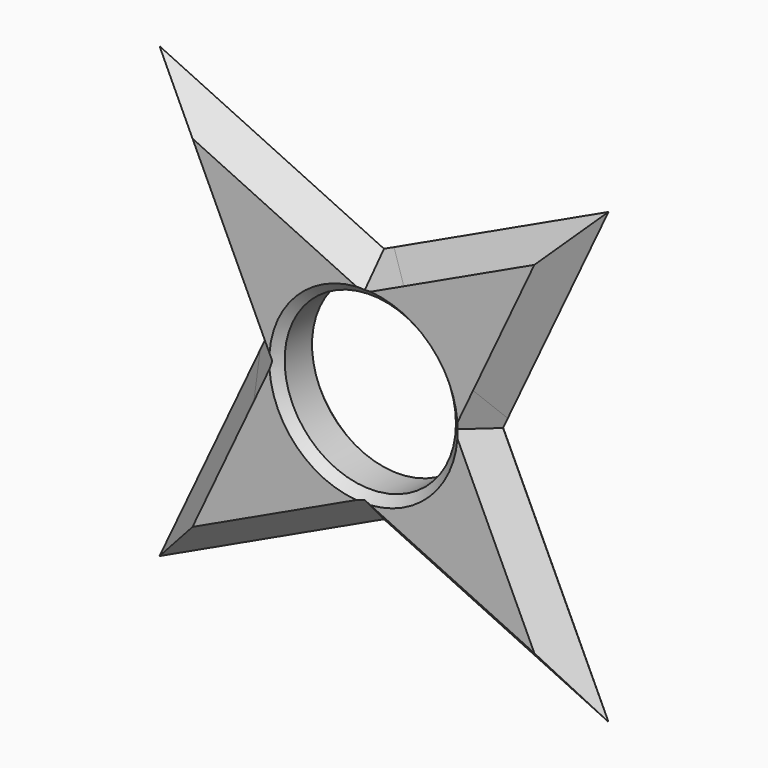
from build123d import *

# Parameters (mm, degrees)
F0_R          = 12.7
F1_DEPTH      = 7.62
F2_SIZE       = 1.27
F3_SIZE       = 1.27
F4_SIZE       = 5.08
F5_T4_DEPTH   = 65.8139573625
F6_SIZE       = 5.08
F7_T4_DEPTH   = 57.8584590231
F8_T4_DEPTH   = 72.4149723957
F8_T10_DEPTH  = 72.4149723957
F8_T16_DEPTH  = 72.4149723957
F9_T4_DEPTH   = 72.4149723957
F10_SIZE      = 5.08
F11_T4_DEPTH  = 57.8584590231
F12_T4_DEPTH  = 72.4149723957
F12_T10_DEPTH = 72.4149723957
F12_T16_DEPTH = 72.4149723957
F13_T4_DEPTH  = 72.4149723957
F14_SIZE      = 5.08
F15_T4_DEPTH  = 57.8584590231
F16_T4_DEPTH  = 72.4149723957
F16_T10_DEPTH = 72.4149723957
F16_T16_DEPTH = 72.4149723957
F17_T4_DEPTH  = 72.4149723957
F18_T4_DEPTH  = 64.4594740563
F18_T10_DEPTH = 64.4594740563
F18_T16_DEPTH = 64.4594740563
F19_T4_DEPTH  = 64.4594740563


# Not quite as in the source:
# - a fillet or chamfer that OpenCascade refuses, or shapes differently, is made with other operations: its cross-section is extruded or revolved along the edge and cut away or added


with BuildPart() as f1:
    # F0 (on Front) → F1 (new body)
    with BuildSketch(Plane.XZ):
        Polygon((-19.05, 0), (-35.9210244843, -35.9210244843), (0, -19.05), (35.9210244843, -35.9210244843), (19.05, 0), (35.9210244843, 35.9210244843), (0, 19.05), (-35.9210244843, 35.9210244843), align=None)
        Circle(F0_R, mode=Mode.SUBTRACT)
    extrude(amount=F1_DEPTH)

    # F2
    f2_edges = [f1.edges().sort_by_distance(p)[0] for p in [
        (-12.7, -7.62, 0),
    ]]
    chamfer(f2_edges, length=F2_SIZE)

    # F3
    f3_edges = [f1.edges().sort_by_distance(p)[0] for p in [
        (-12.7, 0, 0),
    ]]
    chamfer(f3_edges, length=F3_SIZE)

    # F4
    f4_edges = [f1.edges().sort_by_distance(p)[0] for p in [
        (17.960512, -7.62, 27.485512),
    ]]
    chamfer(f4_edges, length=F4_SIZE)

    # F5: chamfer of 5.08 on 1 edges, made by hand


with BuildPart() as f5_tool2:
    # F5_s3 → F5_t4 (new body)
    with BuildSketch(Plane(origin=(55.0761279539, 0, 25.8676002856), x_dir=(0, 1, 0), z_dir=(-0.9051386851, 0, -0.4251164085))):
        Polygon((-5.08, -17.2428919509), (0, -12.1628919509), (0, -17.2428919509), align=None)
    extrude(amount=F5_T4_DEPTH)

    split(bisect_by=Plane(origin=(7.330236298, 0, 15.6072085475), x_dir=(0, 1, 0), z_dir=(0.4251164085, 0, 0.9051386851)), keep=Keep.TOP)


with BuildPart() as f1_1:
    add(f1.part)

    # F5_t1: cut F5_tool2
    add(f5_tool2.part, mode=Mode.SUBTRACT)

    # F6
    f6_edges = [f1_1.edges().sort_by_distance(p)[0] for p in [
        (25.794506, -7.62, 14.360098),
    ]]
    chamfer(f6_edges, length=F6_SIZE)

    # F7: chamfer of 5.08 on 1 edges, made by hand


with BuildPart() as f7_tool2:
    # F7_s3 → F7_t4 (new body)
    with BuildSketch(Plane(origin=(-2.1109928963, 0, -4.4946308736), x_dir=(0, 1, 0), z_dir=(0.4251164085, 0, 0.9051386851))):
        Polygon((-5.08, -17.2428919509), (0, -12.1628919509), (0, -17.2428919509), align=None)
    extrude(amount=F7_T4_DEPTH)

    split(bisect_by=Plane(origin=(15.6072085475, 0, 7.330236298), x_dir=(0, 1, 0), z_dir=(0.9051386851, 0, 0.4251164085)), keep=Keep.TOP)


with BuildPart() as f1_2:
    add(f1_1.part)

    # F7_t1: cut F7_tool2
    add(f7_tool2.part, mode=Mode.SUBTRACT)

    # F8: chamfer of 5.08 on 1 edges, made by hand


with BuildPart() as f8_tool2:
    # F8_s3 → F8_t4 (new body)
    with BuildSketch(Plane(origin=(25.8676002856, 0, -55.0761279539), x_dir=(0, 1, 0), z_dir=(-0.4251164085, 0, 0.9051386851))):
        Polygon((-7.62, -12.1628919509), (-2.54, -17.2428919509), (-7.62, -17.2428919509), align=None)
    extrude(amount=F8_T4_DEPTH)

    split(bisect_by=Plane(origin=(5.5045520136, 6.0814459754, -2.5853224715), x_dir=(-0.741396788, 0.6710669138, 0), z_dir=(0.6400297021, 0.7071067812, -0.3006026952)), keep=Keep.TOP)

    split(bisect_by=Plane(origin=(8.9531304038, -9.8914459754, -4.2050159878), x_dir=(0.741396788, 0.6710669138, 0), z_dir=(0.6400297021, -0.7071067812, -0.3006026952)), keep=Keep.TOP)


with BuildPart() as f1_3:
    add(f1_2.part)

    # F8_t1: cut F8_tool2
    add(f8_tool2.part, mode=Mode.SUBTRACT)


with BuildPart() as f8_tool8:
    # F8_s9 → F8_t10 (new body)
    with BuildSketch(Plane(origin=(25.8676002856, 0, -55.0761279539), x_dir=(0, 1, 0), z_dir=(-0.4251164085, 0, 0.9051386851))):
        Polygon((-7.62, -12.1628919509), (-2.54, -17.2428919509), (-7.62, -17.2428919509), align=None)
    extrude(amount=F8_T10_DEPTH)

    split(bisect_by=Plane(origin=(5.5045520136, 6.0814459754, -2.5853224715), x_dir=(-0.741396788, 0.6710669138, 0), z_dir=(0.6400297021, 0.7071067812, -0.3006026952)), keep=Keep.TOP)

    split(bisect_by=Plane(origin=(8.9531304038, -9.8914459754, -4.2050159878), x_dir=(-0.741396788, -0.6710669138, 0), z_dir=(-0.6400297021, 0.7071067812, 0.3006026952)), keep=Keep.TOP)


with BuildPart() as f1_4:
    add(f1_3.part)

    # F8_t7: cut F8_tool8
    add(f8_tool8.part, mode=Mode.SUBTRACT)


with BuildPart() as f8_tool14:
    # F8_s15 → F8_t16 (new body)
    with BuildSketch(Plane(origin=(25.8676002856, 0, -55.0761279539), x_dir=(0, 1, 0), z_dir=(-0.4251164085, 0, 0.9051386851))):
        Polygon((-7.62, -12.1628919509), (-2.54, -17.2428919509), (-7.62, -17.2428919509), align=None)
    extrude(amount=F8_T16_DEPTH)

    split(bisect_by=Plane(origin=(5.5045520136, 6.0814459754, -2.5853224715), x_dir=(0.741396788, -0.6710669138, 0), z_dir=(-0.6400297021, -0.7071067812, 0.3006026952)), keep=Keep.TOP)

    split(bisect_by=Plane(origin=(8.9531304038, -9.8914459754, -4.2050159878), x_dir=(0.741396788, 0.6710669138, 0), z_dir=(0.6400297021, -0.7071067812, -0.3006026952)), keep=Keep.TOP)


with BuildPart() as f1_5:
    add(f1_4.part)

    # F8_t13: cut F8_tool14
    add(f8_tool14.part, mode=Mode.SUBTRACT)

    # F9: chamfer of 5.08 on 1 edges, made by hand


with BuildPart() as f9_tool2:
    # F9_s3 → F9_t4 (new body)
    with BuildSketch(Plane(origin=(25.8676002856, 0, -55.0761279539), x_dir=(0, 1, 0), z_dir=(-0.4251164085, 0, 0.9051386851))):
        Polygon((0, -12.1628919509), (-5.08, -17.2428919509), (0, -17.2428919509), align=None)
    extrude(amount=F9_T4_DEPTH)

    split(bisect_by=Plane(origin=(5.5045520136, 6.0814459754, -2.5853224715), x_dir=(-0.741396788, 0.6710669138, 0), z_dir=(0.6400297021, 0.7071067812, -0.3006026952)), keep=Keep.TOP)


with BuildPart() as f1_6:
    add(f1_5.part)

    # F9_t1: cut F9_tool2
    add(f9_tool2.part, mode=Mode.SUBTRACT)

    # F10
    f10_edges = [f1_6.edges().sort_by_distance(p)[0] for p in [
        (14.360098, -7.62, -25.794506),
    ]]
    chamfer(f10_edges, length=F10_SIZE)

    # F11: chamfer of 5.08 on 1 edges, made by hand


with BuildPart() as f11_tool2:
    # F11_s3 → F11_t4 (new body)
    with BuildSketch(Plane(origin=(-4.4946308736, 0, 2.1109928963), x_dir=(0, 1, 0), z_dir=(0.9051386851, 0, -0.4251164085))):
        Polygon((-5.08, -17.2428919509), (0, -12.1628919509), (0, -17.2428919509), align=None)
    extrude(amount=F11_T4_DEPTH)

    split(bisect_by=Plane(origin=(7.330236298, 0, -15.6072085475), x_dir=(0, 1, 0), z_dir=(0.4251164085, 0, -0.9051386851)), keep=Keep.TOP)


with BuildPart() as f1_7:
    add(f1_6.part)

    # F11_t1: cut F11_tool2
    add(f11_tool2.part, mode=Mode.SUBTRACT)

    # F12: chamfer of 5.08 on 1 edges, made by hand


with BuildPart() as f12_tool2:
    # F12_s3 → F12_t4 (new body)
    with BuildSketch(Plane(origin=(-55.0761279539, 0, -25.8676002856), x_dir=(0, 1, 0), z_dir=(0.9051386851, 0, 0.4251164085))):
        Polygon((0, -12.1628919509), (-5.08, -17.2428919509), (0, -17.2428919509), align=None)
    extrude(amount=F12_T4_DEPTH)

    split(bisect_by=Plane(origin=(-4.2050159878, -9.8914459754, -8.9531304038), x_dir=(0.9202923495, -0.3912313784, 0), z_dir=(-0.3006026952, -0.7071067812, -0.6400297021)), keep=Keep.TOP)

    split(bisect_by=Plane(origin=(-2.5853224715, 6.0814459755, -5.5045520136), x_dir=(-0.9202923495, -0.3912313784, 0), z_dir=(-0.3006026952, 0.7071067812, -0.6400297021)), keep=Keep.TOP)


with BuildPart() as f1_8:
    add(f1_7.part)

    # F12_t1: cut F12_tool2
    add(f12_tool2.part, mode=Mode.SUBTRACT)


with BuildPart() as f12_tool8:
    # F12_s9 → F12_t10 (new body)
    with BuildSketch(Plane(origin=(-55.0761279539, 0, -25.8676002856), x_dir=(0, 1, 0), z_dir=(0.9051386851, 0, 0.4251164085))):
        Polygon((0, -12.1628919509), (-5.08, -17.2428919509), (0, -17.2428919509), align=None)
    extrude(amount=F12_T10_DEPTH)

    split(bisect_by=Plane(origin=(-4.2050159878, -9.8914459754, -8.9531304038), x_dir=(0.9202923495, -0.3912313784, 0), z_dir=(-0.3006026952, -0.7071067812, -0.6400297021)), keep=Keep.TOP)

    split(bisect_by=Plane(origin=(-2.5853224715, 6.0814459755, -5.5045520136), x_dir=(0.9202923495, 0.3912313784, 0), z_dir=(0.3006026952, -0.7071067812, 0.6400297021)), keep=Keep.TOP)


with BuildPart() as f1_9:
    add(f1_8.part)

    # F12_t7: cut F12_tool8
    add(f12_tool8.part, mode=Mode.SUBTRACT)


with BuildPart() as f12_tool14:
    # F12_s15 → F12_t16 (new body)
    with BuildSketch(Plane(origin=(-55.0761279539, 0, -25.8676002856), x_dir=(0, 1, 0), z_dir=(0.9051386851, 0, 0.4251164085))):
        Polygon((0, -12.1628919509), (-5.08, -17.2428919509), (0, -17.2428919509), align=None)
    extrude(amount=F12_T16_DEPTH)

    split(bisect_by=Plane(origin=(-4.2050159878, -9.8914459754, -8.9531304038), x_dir=(-0.9202923495, 0.3912313784, 0), z_dir=(0.3006026952, 0.7071067812, 0.6400297021)), keep=Keep.TOP)

    split(bisect_by=Plane(origin=(-2.5853224715, 6.0814459755, -5.5045520136), x_dir=(-0.9202923495, -0.3912313784, 0), z_dir=(-0.3006026952, 0.7071067812, -0.6400297021)), keep=Keep.TOP)


with BuildPart() as f1_10:
    add(f1_9.part)

    # F12_t13: cut F12_tool14
    add(f12_tool14.part, mode=Mode.SUBTRACT)

    # F13: chamfer of 5.08 on 1 edges, made by hand


with BuildPart() as f13_tool2:
    # F13_s3 → F13_t4 (new body)
    with BuildSketch(Plane(origin=(-55.0761279539, 0, -25.8676002856), x_dir=(0, 1, 0), z_dir=(0.9051386851, 0, 0.4251164085))):
        Polygon((-7.62, -12.1628919509), (-2.54, -17.2428919509), (-7.62, -17.2428919509), align=None)
    extrude(amount=F13_T4_DEPTH)

    split(bisect_by=Plane(origin=(-4.2050159878, -9.8914459754, -8.9531304038), x_dir=(0.9202923495, -0.3912313784, 0), z_dir=(-0.3006026952, -0.7071067812, -0.6400297021)), keep=Keep.TOP)


with BuildPart() as f1_11:
    add(f1_10.part)

    # F13_t1: cut F13_tool2
    add(f13_tool2.part, mode=Mode.SUBTRACT)

    # F14
    f14_edges = [f1_11.edges().sort_by_distance(p)[0] for p in [
        (-25.794506, -7.62, -14.360098),
    ]]
    chamfer(f14_edges, length=F14_SIZE)

    # F15: chamfer of 5.08 on 1 edges, made by hand


with BuildPart() as f15_tool2:
    # F15_s3 → F15_t4 (new body)
    with BuildSketch(Plane(origin=(2.1109928963, 0, 4.4946308736), x_dir=(0, 1, 0), z_dir=(-0.4251164085, 0, -0.9051386851))):
        Polygon((-5.08, -17.2428919509), (0, -12.1628919509), (0, -17.2428919509), align=None)
    extrude(amount=F15_T4_DEPTH)

    split(bisect_by=Plane(origin=(-15.6072085475, 0, -7.330236298), x_dir=(0, 1, 0), z_dir=(-0.9051386851, 0, -0.4251164085)), keep=Keep.TOP)


with BuildPart() as f1_12:
    add(f1_11.part)

    # F15_t1: cut F15_tool2
    add(f15_tool2.part, mode=Mode.SUBTRACT)

    # F16: chamfer of 5.08 on 1 edges, made by hand


with BuildPart() as f16_tool2:
    # F16_s3 → F16_t4 (new body)
    with BuildSketch(Plane(origin=(-25.8676002856, 0, 55.0761279539), x_dir=(0, 1, 0), z_dir=(0.4251164085, 0, -0.9051386851))):
        Polygon((-7.62, -12.1628919509), (-2.54, -17.2428919509), (-7.62, -17.2428919509), align=None)
    extrude(amount=F16_T4_DEPTH)

    split(bisect_by=Plane(origin=(-5.5045520136, 6.0814459754, 2.5853224715), x_dir=(-0.741396788, -0.6710669138, 0), z_dir=(-0.6400297021, 0.7071067812, 0.3006026952)), keep=Keep.TOP)

    split(bisect_by=Plane(origin=(-8.9531304038, -9.8914459754, 4.2050159878), x_dir=(0.741396788, -0.6710669138, 0), z_dir=(-0.6400297021, -0.7071067812, 0.3006026952)), keep=Keep.TOP)


with BuildPart() as f1_13:
    add(f1_12.part)

    # F16_t1: cut F16_tool2
    add(f16_tool2.part, mode=Mode.SUBTRACT)


with BuildPart() as f16_tool8:
    # F16_s9 → F16_t10 (new body)
    with BuildSketch(Plane(origin=(-25.8676002856, 0, 55.0761279539), x_dir=(0, 1, 0), z_dir=(0.4251164085, 0, -0.9051386851))):
        Polygon((-7.62, -12.1628919509), (-2.54, -17.2428919509), (-7.62, -17.2428919509), align=None)
    extrude(amount=F16_T10_DEPTH)

    split(bisect_by=Plane(origin=(-5.5045520136, 6.0814459754, 2.5853224715), x_dir=(-0.741396788, -0.6710669138, 0), z_dir=(-0.6400297021, 0.7071067812, 0.3006026952)), keep=Keep.TOP)

    split(bisect_by=Plane(origin=(-8.9531304038, -9.8914459754, 4.2050159878), x_dir=(-0.741396788, 0.6710669138, 0), z_dir=(0.6400297021, 0.7071067812, -0.3006026952)), keep=Keep.TOP)


with BuildPart() as f1_14:
    add(f1_13.part)

    # F16_t7: cut F16_tool8
    add(f16_tool8.part, mode=Mode.SUBTRACT)


with BuildPart() as f16_tool14:
    # F16_s15 → F16_t16 (new body)
    with BuildSketch(Plane(origin=(-25.8676002856, 0, 55.0761279539), x_dir=(0, 1, 0), z_dir=(0.4251164085, 0, -0.9051386851))):
        Polygon((-7.62, -12.1628919509), (-2.54, -17.2428919509), (-7.62, -17.2428919509), align=None)
    extrude(amount=F16_T16_DEPTH)

    split(bisect_by=Plane(origin=(-5.5045520136, 6.0814459754, 2.5853224715), x_dir=(0.741396788, 0.6710669138, 0), z_dir=(0.6400297021, -0.7071067812, -0.3006026952)), keep=Keep.TOP)

    split(bisect_by=Plane(origin=(-8.9531304038, -9.8914459754, 4.2050159878), x_dir=(0.741396788, -0.6710669138, 0), z_dir=(-0.6400297021, -0.7071067812, 0.3006026952)), keep=Keep.TOP)


with BuildPart() as f1_15:
    add(f1_14.part)

    # F16_t13: cut F16_tool14
    add(f16_tool14.part, mode=Mode.SUBTRACT)

    # F17: chamfer of 5.08 on 1 edges, made by hand


with BuildPart() as f17_tool2:
    # F17_s3 → F17_t4 (new body)
    with BuildSketch(Plane(origin=(4.9171926996, 0, -10.4694649409), x_dir=(0, 1, 0), z_dir=(-0.4251164085, 0, 0.9051386851))):
        Polygon((-5.08, 17.2428919509), (0, 12.1628919509), (0, 17.2428919509), align=None)
    extrude(amount=F17_T4_DEPTH)

    split(bisect_by=Plane(origin=(-5.5045520136, 6.0814459754, 2.5853224715), x_dir=(-0.741396788, -0.6710669138, 0), z_dir=(-0.6400297021, 0.7071067812, 0.3006026952)), keep=Keep.TOP)


with BuildPart() as f1_16:
    add(f1_15.part)

    # F17_t1: cut F17_tool2
    add(f17_tool2.part, mode=Mode.SUBTRACT)

    # F18: chamfer of 5.08 on 1 edges, made by hand


with BuildPart() as f18_tool2:
    # F18_s3 → F18_t4 (new body)
    with BuildSketch(Plane(origin=(10.469464941, 0, -4.9171926996), x_dir=(0, 1, 0), z_dir=(-0.9051386851, 0, 0.4251164085))):
        Polygon((-2.54, -17.2428919509), (-7.62, -12.1628919509), (-7.62, -17.2428919509), align=None)
    extrude(amount=F18_T4_DEPTH)

    split(bisect_by=Plane(origin=(-4.2050159878, -9.8914459754, 8.9531304038), x_dir=(0.9202923495, -0.3912313784, 0), z_dir=(-0.3006026952, -0.7071067812, 0.6400297021)), keep=Keep.TOP)

    split(bisect_by=Plane(origin=(-2.5853224715, 6.0814459755, 5.5045520136), x_dir=(0.9202923495, 0.3912313784, 0), z_dir=(0.3006026952, -0.7071067812, -0.6400297021)), keep=Keep.TOP)


with BuildPart() as f1_17:
    add(f1_16.part)

    # F18_t1: cut F18_tool2
    add(f18_tool2.part, mode=Mode.SUBTRACT)


with BuildPart() as f18_tool8:
    # F18_s9 → F18_t10 (new body)
    with BuildSketch(Plane(origin=(10.469464941, 0, -4.9171926996), x_dir=(0, 1, 0), z_dir=(-0.9051386851, 0, 0.4251164085))):
        Polygon((-2.54, -17.2428919509), (-7.62, -12.1628919509), (-7.62, -17.2428919509), align=None)
    extrude(amount=F18_T10_DEPTH)

    split(bisect_by=Plane(origin=(-4.2050159878, -9.8914459754, 8.9531304038), x_dir=(-0.9202923495, 0.3912313784, 0), z_dir=(0.3006026952, 0.7071067812, -0.6400297021)), keep=Keep.TOP)

    split(bisect_by=Plane(origin=(-2.5853224715, 6.0814459755, 5.5045520136), x_dir=(-0.9202923495, -0.3912313784, 0), z_dir=(-0.3006026952, 0.7071067812, 0.6400297021)), keep=Keep.TOP)


with BuildPart() as f1_18:
    add(f1_17.part)

    # F18_t7: cut F18_tool8
    add(f18_tool8.part, mode=Mode.SUBTRACT)


with BuildPart() as f18_tool14:
    # F18_s15 → F18_t16 (new body)
    with BuildSketch(Plane(origin=(10.469464941, 0, -4.9171926996), x_dir=(0, 1, 0), z_dir=(-0.9051386851, 0, 0.4251164085))):
        Polygon((-2.54, -17.2428919509), (-7.62, -12.1628919509), (-7.62, -17.2428919509), align=None)
    extrude(amount=F18_T16_DEPTH)

    split(bisect_by=Plane(origin=(-4.2050159878, -9.8914459754, 8.9531304038), x_dir=(0.9202923495, -0.3912313784, 0), z_dir=(-0.3006026952, -0.7071067812, 0.6400297021)), keep=Keep.TOP)

    split(bisect_by=Plane(origin=(-2.5853224715, 6.0814459755, 5.5045520136), x_dir=(-0.9202923495, -0.3912313784, 0), z_dir=(-0.3006026952, 0.7071067812, 0.6400297021)), keep=Keep.TOP)


with BuildPart() as f1_19:
    add(f1_18.part)

    # F18_t13: cut F18_tool14
    add(f18_tool14.part, mode=Mode.SUBTRACT)

    # F19: chamfer of 5.08 on 1 edges, made by hand


with BuildPart() as f19_tool2:
    # F19_s3 → F19_t4 (new body)
    with BuildSketch(Plane(origin=(10.4694649409, 0, -4.9171926996), x_dir=(0, 1, 0), z_dir=(-0.9051386851, 0, 0.4251164085))):
        Polygon((-5.08, -17.2428919509), (0, -12.1628919509), (0, -17.2428919509), align=None)
    extrude(amount=F19_T4_DEPTH)

    split(bisect_by=Plane(origin=(-2.5853224715, 6.0814459755, 5.5045520136), x_dir=(-0.9202923495, -0.3912313784, 0), z_dir=(-0.3006026952, 0.7071067812, 0.6400297021)), keep=Keep.TOP)


with BuildPart() as f1_20:
    add(f1_19.part)

    # F19_t1: cut F19_tool2
    add(f19_tool2.part, mode=Mode.SUBTRACT)


solid = f1_20.part
